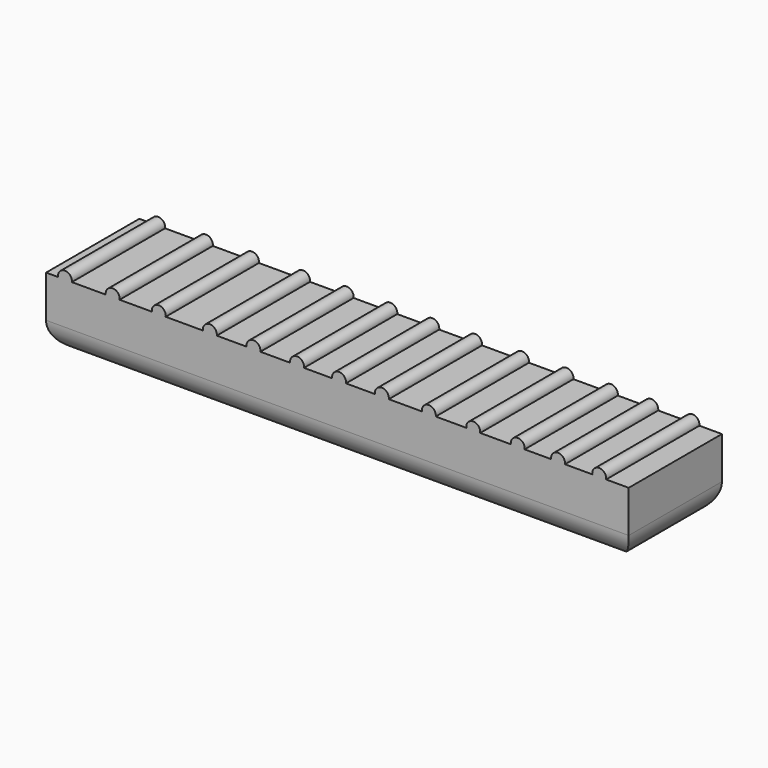
from build123d import *

# Parameters (mm, degrees)
F0_W          = 158.75
F0_H          = 31.75
F1_DEPTH      = 19.05
F3_R          = 7.62
F2_R          = 1.905
F4_DEPTH      = 21.9981725439
F4_DEPTH_BACK = 9.7518274561


with BuildPart() as f1:
    # F0 (on Top) → F1 (new body)
    with BuildSketch(Plane.XY):
        with Locations((-43.8790681958, 6.1231725439)):
            Rectangle(F0_W, F0_H)
    extrude(amount=F1_DEPTH)

    # F3
    f3_edges = [f1.edges().sort_by_distance(p)[0] for p in [
        (-43.879068, 21.998173, 0),
        (-123.254068, 6.123173, 0),
        (-43.879068, -9.751827, 0),
        (35.495932, 6.123173, 0),
    ]]
    fillet(f3_edges, radius=F3_R)

    # F2 (on Front) → F4 (join, two sides)
    with BuildSketch(Plane.XZ) as f4_sk:
        with Locations((-105.110168457, 19.2852988839)):
            Circle(F2_R)
        with Locations((-92.5481468439, 19.2852988839)):
            Circle(F2_R)
        with Locations((-78.6401927471, 19.2852988839)):
            Circle(F2_R)
        with Locations((-66.7505128102, 19.2852988839)):
            Circle(F2_R)
        with Locations((-54.8614611642, 19.2852988839)):
            Circle(F2_R)
        with Locations((-43.4210499542, 19.2852988839)):
            Circle(F2_R)
        with Locations((-31.7563166635, 19.2852988839)):
            Circle(F2_R)
        with Locations((-18.9705938101, 19.2852988839)):
            Circle(F2_R)
        with Locations((-6.8572163582, 19.2852988839)):
            Circle(F2_R)
        with Locations((-118.1202022152, 19.2852988839)):
            Circle(F2_R)
        with Locations((5.2561564371, 19.2852988839)):
            Circle(F2_R)
        with Locations((16.2479281425, 19.2852988839)):
            Circle(F2_R)
        with Locations((27.4640191346, 19.2852988839)):
            Circle(F2_R)
    extrude(amount=-F4_DEPTH)
    extrude(f4_sk.sketch, amount=F4_DEPTH_BACK)


solid = f1.part
